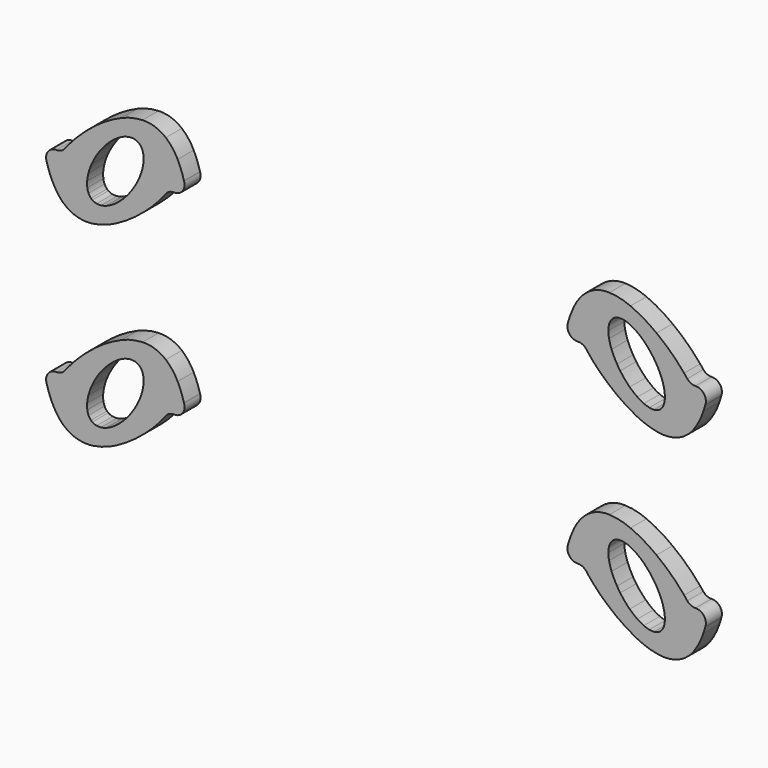
from build123d import *

# Parameters (mm, degrees)
F1_DEPTH = 12.7


# Not quite as in the source:
# - ends of sketch curves that miss each other by under 0.0002 mm in the source are joined


with BuildPart() as f1:
    # F0 (on Front) → F1 (new body)
    with BuildSketch(Plane.XZ):
        with BuildLine():
            ThreePointArc((-177.6953938627, 96.2951726391), (-186.946967119, 88.4805061313), (-195.2020417923, 79.6196730731))
            Line((-195.2020417923, 79.6196730731), (-197.2011042, 77.1213088))
            ThreePointArc((-197.2011042, 77.1213088), (-199.5136578752, 75.3159529873), (-202.3909333919, 74.7428131786))
            ThreePointArc((-202.3909333919, 74.7428131786), (-207.7133187116, 72.1927198012), (-208.6383219414, 66.3638994003))
            Line((-208.6383219414, 66.3638994003), (-208.5382926, 66.0395936))
            ThreePointArc((-208.5382926, 66.0395936), (-207.972327333, 64.1185028331), (-207.353315885, 62.2138423713))
            ThreePointArc((-207.353315885, 62.2138423713), (-204.7701961443, 55.9663745774), (-201.2342339233, 50.2044021579))
            ThreePointArc((-201.2342339233, 50.2044021579), (-196.8863760333, 45.6616875081), (-191.4694434874, 42.4684149565))
            Line((-191.4694434874, 42.4684149565), (-191.284098, 42.3952924))
            ThreePointArc((-191.284098, 42.3952924), (-185.1027368685, 40.9837502599), (-178.7669800767, 41.2283522882))
            ThreePointArc((-178.7669800767, 41.2283522882), (-171.6181643219, 43.0302257906), (-164.8462206323, 45.9445209219))
            ThreePointArc((-164.8462206323, 45.9445209219), (-155.3582667886, 51.6671412258), (-146.6297283987, 58.4922616416))
            ThreePointArc((-146.6297283987, 58.4922616416), (-139.9244707914, 64.8347082096), (-133.9056606053, 71.8319248327))
            Line((-133.9056606053, 71.8319248327), (-133.2299342, 72.7382086))
            ThreePointArc((-133.2299342, 72.7382086), (-130.8614812662, 74.6793213027), (-127.8599677834, 75.2862607769))
            ThreePointArc((-127.8599677834, 75.2862607769), (-122.5270410705, 77.7851692011), (-121.5411283463, 83.5914271061))
            Line((-121.5411283463, 83.5914271061), (-121.6296272, 83.8884276))
            ThreePointArc((-121.6296272, 83.8884276), (-123.378440433, 89.2760477142), (-125.6424834839, 94.468245494))
            ThreePointArc((-125.6424834839, 94.468245494), (-128.8762830329, 99.7114239774), (-133.1072855129, 104.1888096209))
            ThreePointArc((-133.1072855129, 104.1888096209), (-140.0332321267, 108.0332940551), (-147.8805780907, 109.1140330857))
            ThreePointArc((-147.8805780907, 109.1140330857), (-154.6765471368, 108.1634211001), (-161.1886536518, 105.9997872024))
            ThreePointArc((-161.1886536518, 105.9997872024), (-169.7449307333, 101.6626983872), (-177.6953938627, 96.2951726391))
        make_face()
        with BuildLine():
            ThreePointArc((-176.9480341869, 53.1001419638), (-178.3700174028, 53.5041929641), (-179.6704836172, 54.2071019928))
            ThreePointArc((-179.6704836172, 54.2071019928), (-180.120026778, 54.5527599218), (-180.5373020377, 54.9367507345))
            ThreePointArc((-180.5373020377, 54.9367507345), (-181.3997214321, 55.9967169239), (-182.0537255517, 57.1965381674))
            ThreePointArc((-182.0537255517, 57.1965381674), (-182.5422088404, 58.5758677997), (-182.8412153057, 60.0082653866))
            ThreePointArc((-182.8412153057, 60.0082653866), (-182.996770745, 61.812213744), (-182.9585847837, 63.6224550888))
            ThreePointArc((-182.9585847837, 63.6224550888), (-182.6792234379, 65.9600035096), (-182.1897058816, 68.2627290379))
            ThreePointArc((-182.1897058816, 68.2627290379), (-181.2724223103, 71.2729875245), (-180.1069387677, 74.1961219073))
            ThreePointArc((-180.1069387677, 74.1961219073), (-178.0007024043, 78.3577185897), (-175.5048634466, 82.2980118343))
            ThreePointArc((-175.5048634466, 82.2980118343), (-174.4173435256, 83.792470291), (-173.2758101811, 85.2460890182))
            ThreePointArc((-173.2758101811, 85.2460890182), (-170.6569263411, 88.2024335216), (-167.7913192063, 90.920303724))
            ThreePointArc((-167.7913192063, 90.920303724), (-165.5649042541, 92.6984257891), (-163.19628366, 94.2821808259))
            ThreePointArc((-163.19628366, 94.2821808259), (-161.2999842726, 95.3190481003), (-159.3137266172, 96.1710013699))
            ThreePointArc((-159.3137266172, 96.1710013699), (-157.7154103749, 96.6676730685), (-156.0708086919, 96.9784499128))
            ThreePointArc((-156.0708086919, 96.9784499128), (-154.6610921749, 97.057810869), (-153.2552179199, 96.9269846745))
            ThreePointArc((-153.2552179199, 96.9269846745), (-151.8332434746, 96.5229429708), (-150.5327847695, 95.8200418883))
            ThreePointArc((-150.5327847695, 95.8200418883), (-150.0832461196, 95.4743903416), (-149.6659744937, 95.0904067336))
            ThreePointArc((-149.6659744937, 95.0904067336), (-148.8035282211, 94.0304381711), (-148.1495164134, 92.8305978145))
            ThreePointArc((-148.1495164134, 92.8305978145), (-147.6610428325, 91.4512658888), (-147.3620363785, 90.0188700866))
            ThreePointArc((-147.3620363785, 90.0188700866), (-147.2065050667, 88.2149193747), (-147.2446935639, 86.4046789413))
            ThreePointArc((-147.2446935639, 86.4046789413), (-147.5240277621, 84.0671284904), (-148.0135453184, 81.7644029621))
            ThreePointArc((-148.0135453184, 81.7644029621), (-148.9308288897, 78.7541444755), (-150.0963124323, 75.8310100927))
            ThreePointArc((-150.0963124323, 75.8310100927), (-152.2025628964, 71.6694333025), (-154.6983928041, 67.7291491159))
            ThreePointArc((-154.6983928041, 67.7291491159), (-155.7859116303, 66.2346900702), (-156.927443836, 64.7810706787))
            ThreePointArc((-156.927443836, 64.7810706787), (-159.5463306489, 61.8247178881), (-162.4119445698, 59.1068427459))
            ThreePointArc((-162.4119445698, 59.1068427459), (-164.6383679218, 57.3287348477), (-167.0069856984, 55.7449809851))
            ThreePointArc((-167.0069856984, 55.7449809851), (-168.9032728768, 54.7081064054), (-170.8895245828, 53.8561560301))
            ThreePointArc((-170.8895245828, 53.8561560301), (-172.487848721, 53.3594569655), (-174.1324674845, 53.0486788344))
            ThreePointArc((-174.1324674845, 53.0486788344), (-175.5421719045, 52.9693209022), (-176.9480341869, 53.1001419638))
        make_face(mode=Mode.SUBTRACT)
    extrude(amount=F1_DEPTH)


with BuildPart() as f1b:
    # F0 (on Front) → F1, piece 2 (new body)
    with BuildSketch(Plane.XZ):
        with BuildLine():
            Line((197.2011042, -46.6997796), (195.2020734, -44.2014102))
            ThreePointArc((195.2020734, -44.2014102), (186.9469729749, -35.3405878466), (177.6953938627, -27.5259157609))
            ThreePointArc((177.6953938627, -27.5259157609), (169.7449307333, -22.1583900128), (161.1886562004, -17.8212952927))
            ThreePointArc((161.1886562004, -17.8212952927), (154.6765477311, -15.6576674389), (147.8805787114, -14.7070678147))
            ThreePointArc((147.8805787114, -14.7070678147), (140.033241985, -15.7877910583), (133.1072927899, -19.6322572713))
            ThreePointArc((133.1072927899, -19.6322572713), (128.8762888916, -24.1096567935), (125.6424960866, -29.3528491583))
            ThreePointArc((125.6424960866, -29.3528491583), (123.3784626535, -34.5450490683), (121.629632462, -39.9326622292))
            Line((121.629632462, -39.9326622292), (121.5411336, -40.229663))
            ThreePointArc((121.5411336, -40.229663), (122.5270410705, -46.0359191989), (127.8599678166, -48.5348283769))
            ThreePointArc((127.8599678166, -48.5348283769), (130.8614904645, -49.141771462), (133.2299305689, -51.0829079075))
            Line((133.2299305689, -51.0829079075), (133.9056758, -51.9891518))
            ThreePointArc((133.9056758, -51.9891518), (139.9244908242, -58.9863745636), (146.6297484323, -65.3288331002))
            ThreePointArc((146.6297484323, -65.3288331002), (155.3582746235, -72.153952571), (164.8462212522, -77.8765664355))
            ThreePointArc((164.8462212522, -77.8765664355), (171.6181672262, -80.7908549881), (178.7669774619, -82.5927513887))
            ThreePointArc((178.7669774619, -82.5927513887), (185.1027368685, -82.8373381401), (191.2840912155, -81.4257777575))
            Line((191.2840912155, -81.4257777575), (191.4694418, -81.3526694))
            ThreePointArc((191.4694418, -81.3526694), (196.8863760333, -78.1594008919), (201.2342450386, -73.6166943298))
            ThreePointArc((201.2342450386, -73.6166943298), (204.7701906585, -67.854724589), (207.3533009369, -61.6072664326))
            ThreePointArc((207.3533009369, -61.6072664326), (207.9723237758, -59.7025970512), (208.5382965738, -57.7814959111))
            Line((208.5382965738, -57.7814959111), (208.6383432, -57.4571876))
            ThreePointArc((208.6383432, -57.4571876), (207.7133441116, -51.6283685988), (202.390958682, -49.0782722124))
            ThreePointArc((202.390958682, -49.0782722124), (199.5136608193, -48.505162162), (197.2011042, -46.6997796))
        make_face()
        with BuildLine():
            ThreePointArc((181.6418108826, -67.4343387272), (180.7757849638, -68.6323663846), (179.6704878904, -69.6139923518))
            ThreePointArc((179.6704878904, -69.6139923518), (179.1919244089, -69.9182129674), (178.6883710607, -70.1789938892))
            ThreePointArc((178.6883710607, -70.1789938892), (177.3973595426, -70.6268807263), (176.046206417, -70.8310787354))
            ThreePointArc((176.046206417, -70.8310787354), (174.582987936, -70.8183379879), (173.1347072073, -70.6094026153))
            ThreePointArc((173.1347072073, -70.6094026153), (171.3863477646, -70.1385669414), (169.6983350536, -69.4835393235))
            ThreePointArc((169.6983350536, -69.4835393235), (167.5973067728, -68.4215563874), (165.6008854485, -67.1739866994))
            ThreePointArc((165.6008854485, -67.1739866994), (163.0858995952, -65.2824509498), (160.7376709293, -63.1874846573))
            ThreePointArc((160.7376709293, -63.1874846573), (157.5474251459, -59.7849217056), (154.6983881005, -56.091942552))
            ThreePointArc((154.6983881005, -56.091942552), (153.666026198, -54.5588585969), (152.6904970156, -52.9889990603))
            ThreePointArc((152.6904970156, -52.9889990603), (150.8081304363, -49.5169353174), (149.2342629952, -45.8945772719))
            ThreePointArc((149.2342629952, -45.8945772719), (148.3248710619, -43.1942704045), (147.6467445575, -40.4268180092))
            ThreePointArc((147.6467445575, -40.4268180092), (147.3209800199, -38.2902606469), (147.1997449811, -36.1324142807))
            ThreePointArc((147.1997449811, -36.1324142807), (147.2796619641, -34.4606010377), (147.5501168773, -32.8088736105))
            ThreePointArc((147.5501168773, -32.8088736105), (147.9577088343, -31.4570460365), (148.5614749513, -30.1807113181))
            ThreePointArc((148.5614749513, -30.1807113181), (149.4274916362, -28.9826784154), (150.5327887096, -28.0010524482))
            ThreePointArc((150.5327887096, -28.0010524482), (151.0113422017, -27.6968375795), (151.5148846236, -27.4360605956))
            ThreePointArc((151.5148846236, -27.4360605956), (152.8059065439, -26.9881666685), (154.1570716534, -26.7839659792))
            ThreePointArc((154.1570716534, -26.7839659792), (155.6202894054, -26.7967068686), (157.0685693927, -27.0056421847))
            ThreePointArc((157.0685693927, -27.0056421847), (158.8169128719, -27.4764726285), (160.5049109204, -28.1314916634))
            ThreePointArc((160.5049109204, -28.1314916634), (162.6059551987, -29.1934801671), (164.6023911515, -30.4410581006))
            ThreePointArc((164.6023911515, -30.4410581006), (167.1173770048, -32.3325938502), (169.4656056707, -34.4275601427))
            ThreePointArc((169.4656056707, -34.4275601427), (172.6558467449, -37.8301175616), (175.5048801864, -41.5230903297))
            ThreePointArc((175.5048801864, -41.5230903297), (176.5372520953, -43.05616342), (177.5127795844, -44.6260203397))
            ThreePointArc((177.5127795844, -44.6260203397), (179.3951308102, -48.0981047048), (180.9689999614, -51.7204727638))
            ThreePointArc((180.9689999614, -51.7204727638), (181.8784020662, -54.4207624375), (182.556527143, -57.1882023739))
            ThreePointArc((182.556527143, -57.1882023739), (182.8822978837, -59.3247712766), (183.0035318338, -61.4826303007))
            ThreePointArc((183.0035318338, -61.4826303007), (182.9236130271, -63.1544336228), (182.6531585177, -64.8061511889))
            ThreePointArc((182.6531585177, -64.8061511889), (182.2455712306, -66.1579897591), (181.6418108826, -67.4343387272))
        make_face(mode=Mode.SUBTRACT)
    extrude(amount=F1_DEPTH)


with BuildPart() as f1c:
    # F0 (on Front) → F1, piece 3 (new body)
    with BuildSketch(Plane.XZ):
        with BuildLine():
            Line((197.2011042, 77.1213088), (195.202048, 79.6196782))
            ThreePointArc((195.202048, 79.6196782), (186.946967119, 88.4805061313), (177.6953938627, 96.2951726391))
            ThreePointArc((177.6953938627, 96.2951726391), (169.7449307333, 101.6626983872), (161.1886562004, 105.9997931073))
            ThreePointArc((161.1886562004, 105.9997931073), (154.6765471368, 108.1634211001), (147.8805774921, 109.114020644))
            ThreePointArc((147.8805774921, 109.114020644), (140.0332321267, 108.0332940551), (133.1072777232, 104.1888186512))
            ThreePointArc((133.1072777232, 104.1888186512), (128.8762830329, 99.7114239774), (125.6424960866, 94.4682392417))
            ThreePointArc((125.6424960866, 94.4682392417), (123.378440433, 89.2760477142), (121.6296088071, 83.8884325957))
            Line((121.6296088071, 83.8884325957), (121.5411336, 83.5914254))
            ThreePointArc((121.5411336, 83.5914254), (122.5270410705, 77.7851692011), (127.8599678166, 75.2862600231))
            ThreePointArc((127.8599678166, 75.2862600231), (130.8614812662, 74.6793213027), (133.229918397, 72.7381968166))
            Line((133.229918397, 72.7381968166), (133.9056758, 71.8319366))
            ThreePointArc((133.9056758, 71.8319366), (139.9244707914, 64.8347082096), (146.6297230323, 58.4922552998))
            ThreePointArc((146.6297230323, 58.4922552998), (155.3582667886, 51.6671412258), (164.8462212522, 45.9445219645))
            ThreePointArc((164.8462212522, 45.9445219645), (171.6181643219, 43.0302257906), (178.7669767587, 41.2283328438))
            ThreePointArc((178.7669767587, 41.2283328438), (185.1027368685, 40.9837502599), (191.2840912155, 42.3953106425))
            Line((191.2840912155, 42.3953106425), (191.4694418, 42.468419))
            ThreePointArc((191.4694418, 42.468419), (196.8863760333, 45.6616875081), (201.2342450386, 50.2043940702))
            ThreePointArc((201.2342450386, 50.2043940702), (204.7701961443, 55.9663745774), (207.3533083756, 62.2138449609))
            ThreePointArc((207.3533083756, 62.2138449609), (207.972327333, 64.1185028331), (208.5382965738, 66.0395924889))
            Line((208.5382965738, 66.0395924889), (208.6383178, 66.3639008))
            ThreePointArc((208.6383178, 66.3639008), (207.7133187116, 72.1927198012), (202.390933282, 74.7428161876))
            ThreePointArc((202.390933282, 74.7428161876), (199.5136578752, 75.3159529873), (197.2011042, 77.1213088))
        make_face()
        with BuildLine():
            ThreePointArc((181.6418108826, 56.3867496728), (180.7757849638, 55.1887220154), (179.6704878904, 54.2070960482))
            ThreePointArc((179.6704878904, 54.2070960482), (179.1919134729, 53.9028945411), (178.6883613761, 53.6421154265))
            ThreePointArc((178.6883613761, 53.6421154265), (177.3973576804, 53.1942134829), (176.0462063316, 52.9900111351))
            ThreePointArc((176.0462063316, 52.9900111351), (174.582987936, 53.0027504121), (173.1347072073, 53.2116857847))
            ThreePointArc((173.1347072073, 53.2116857847), (171.3863451709, 53.6825139865), (169.6983307601, 54.3375395569))
            ThreePointArc((169.6983307601, 54.3375395569), (167.5973067728, 55.3995320126), (165.6008854485, 56.6471017006))
            ThreePointArc((165.6008854485, 56.6471017006), (163.0858995952, 58.5386374502), (160.7376709293, 60.6336037427))
            ThreePointArc((160.7376709293, 60.6336037427), (157.5474251459, 64.0361666944), (154.6983881005, 67.729145848))
            ThreePointArc((154.6983881005, 67.729145848), (153.6660082898, 69.2622182257), (152.6904782782, 70.8320781665))
            ThreePointArc((152.6904782782, 70.8320781665), (150.8081304363, 74.3041530826), (149.2342629952, 77.9265111281))
            ThreePointArc((149.2342629952, 77.9265111281), (148.3248710619, 80.6268179955), (147.6467445575, 83.3942703908))
            ThreePointArc((147.6467445575, 83.3942703908), (147.3209548909, 85.5308251494), (147.1997195829, 87.6886739026))
            ThreePointArc((147.1997195829, 87.6886739026), (147.2796619641, 89.3604873623), (147.5501168773, 91.0122147895))
            ThreePointArc((147.5501168773, 91.0122147895), (147.957686674, 92.3640507825), (148.5614557429, 93.6403879874))
            ThreePointArc((148.5614557429, 93.6403879874), (149.4274916362, 94.8384099846), (150.5327887096, 95.8200359518))
            ThreePointArc((150.5327887096, 95.8200359518), (151.0113468271, 96.1242534816), (151.5148943083, 96.3850322888))
            ThreePointArc((151.5148943083, 96.3850322888), (152.805911638, 96.8329229888), (154.1570716534, 97.0371224208))
            ThreePointArc((154.1570716534, 97.0371224208), (155.6202770217, 97.0243824743), (157.0685451022, 96.8154514068))
            ThreePointArc((157.0685451022, 96.8154514068), (158.8169010671, 96.3446196392), (160.5049109204, 95.6895967366))
            ThreePointArc((160.5049109204, 95.6895967366), (162.6059551987, 94.6276082329), (164.6023911515, 93.3800302994))
            ThreePointArc((164.6023911515, 93.3800302994), (167.1173894145, 91.4885097773), (169.4656183649, 89.3935413416))
            ThreePointArc((169.4656183649, 89.3935413416), (172.6558252148, 85.9909662917), (175.5048511812, 82.2980032389))
            ThreePointArc((175.5048511812, 82.2980032389), (176.5372464439, 80.7649337135), (177.5127795844, 79.1950680603))
            ThreePointArc((177.5127795844, 79.1950680603), (179.3951288175, 75.7229877857), (180.968996701, 72.1006241323))
            ThreePointArc((180.968996701, 72.1006241323), (181.8784007951, 69.4003303401), (182.556527143, 66.6328860261))
            ThreePointArc((182.556527143, 66.6328860261), (182.8822978837, 64.4963171234), (183.0035318338, 62.3384580993))
            ThreePointArc((183.0035318338, 62.3384580993), (182.9235879044, 60.6666574083), (182.6531343227, 59.0149426105))
            ThreePointArc((182.6531343227, 59.0149426105), (182.2455628115, 57.6631021621), (181.6418108826, 56.3867496728))
        make_face(mode=Mode.SUBTRACT)
    extrude(amount=F1_DEPTH)


with BuildPart() as f1d:
    # F0 (on Front) → F1, piece 4 (new body)
    with BuildSketch(Plane.XZ):
        with BuildLine():
            ThreePointArc((-177.6953938627, -27.5259157609), (-186.9469729749, -35.3405878466), (-195.2020520922, -44.2014277981))
            Line((-195.2020520922, -44.2014277981), (-197.2011042, -46.6997796))
            ThreePointArc((-197.2011042, -46.6997796), (-199.5136608193, -48.505162162), (-202.3909596842, -49.0782996615))
            ThreePointArc((-202.3909596842, -49.0782996615), (-207.7133441116, -51.6283685988), (-208.6383473414, -57.4571889997))
            Line((-208.6383473414, -57.4571889997), (-208.5382926, -57.7814948))
            ThreePointArc((-208.5382926, -57.7814948), (-207.9723237758, -59.7025970512), (-207.3533081368, -61.6072687912))
            ThreePointArc((-207.3533081368, -61.6072687912), (-204.7701906585, -67.854724589), (-201.2342339233, -73.6166862421))
            ThreePointArc((-201.2342339233, -73.6166862421), (-196.8863760333, -78.1594008919), (-191.4694434874, -81.3526734435))
            Line((-191.4694434874, -81.3526734435), (-191.284098, -81.425796))
            ThreePointArc((-191.284098, -81.425796), (-185.1027368685, -82.8373381401), (-178.7669800767, -82.5927361118))
            ThreePointArc((-178.7669800767, -82.5927361118), (-171.6181672262, -80.7908549881), (-164.8462261767, -77.8765569859))
            ThreePointArc((-164.8462261767, -77.8765569859), (-155.3582746235, -72.153952571), (-146.6297426525, -65.328839363))
            ThreePointArc((-146.6297426525, -65.328839363), (-139.9244908242, -58.9863745636), (-133.9056764828, -51.9891512712))
            Line((-133.9056764828, -51.9891512712), (-133.2299342, -51.0829052))
            ThreePointArc((-133.2299342, -51.0829052), (-130.8614904645, -49.141771462), (-127.8599677834, -48.5348276231))
            ThreePointArc((-127.8599677834, -48.5348276231), (-122.5270410705, -46.0359191989), (-121.5411283463, -40.2296612939))
            Line((-121.5411283463, -40.2296612939), (-121.6296272, -39.9326608))
            ThreePointArc((-121.6296272, -39.9326608), (-123.3784626535, -34.5450490683), (-125.6425038809, -29.3528530078))
            ThreePointArc((-125.6425038809, -29.3528530078), (-128.8762888916, -24.1096567935), (-133.1073000843, -19.6322662178))
            ThreePointArc((-133.1073000843, -19.6322662178), (-140.033241985, -15.7877910583), (-147.8805793101, -14.707055373))
            ThreePointArc((-147.8805793101, -14.707055373), (-154.6765477311, -15.6576674389), (-161.1886536518, -17.8213011976))
            ThreePointArc((-161.1886536518, -17.8213011976), (-169.7449307333, -22.1583900128), (-177.6953938627, -27.5259157609))
        make_face()
        with BuildLine():
            ThreePointArc((-176.9480341869, -70.7209464362), (-178.3700174028, -70.3168954359), (-179.6704836172, -69.6139864072))
            ThreePointArc((-179.6704836172, -69.6139864072), (-180.1200373693, -69.2683409431), (-180.5373148061, -68.8843503653))
            ThreePointArc((-180.5373148061, -68.8843503653), (-181.3997418805, -67.8243788549), (-182.0537509517, -66.6245502326))
            ThreePointArc((-182.0537509517, -66.6245502326), (-182.5422101983, -65.245215752), (-182.8412153057, -63.8128230134))
            ThreePointArc((-182.8412153057, -63.8128230134), (-182.996771564, -62.0088748281), (-182.9585828949, -60.1986334524))
            ThreePointArc((-182.9585828949, -60.1986334524), (-182.6792234379, -57.8610848904), (-182.1897058816, -55.5583593621))
            ThreePointArc((-182.1897058816, -55.5583593621), (-181.2724223103, -52.5481008755), (-180.1069387677, -49.6249664927))
            ThreePointArc((-180.1069387677, -49.6249664927), (-178.000707536, -45.4633788446), (-175.5048753963, -41.5230935661))
            ThreePointArc((-175.5048753963, -41.5230935661), (-174.4173498004, -40.0286264079), (-173.2758101811, -38.5749993818))
            ThreePointArc((-173.2758101811, -38.5749993818), (-170.6569268744, -35.6186545514), (-167.7913175603, -32.9007865699))
            ThreePointArc((-167.7913175603, -32.9007865699), (-165.5649130077, -31.1226690154), (-163.1963021863, -29.5389188588))
            ThreePointArc((-163.1963021863, -29.5389188588), (-161.2999980181, -28.5020469868), (-159.3137349454, -27.650090142))
            ThreePointArc((-159.3137349454, -27.650090142), (-157.7154146996, -27.1534164083), (-156.0708086919, -26.8426384872))
            ThreePointArc((-156.0708086919, -26.8426384872), (-154.6610921749, -26.763277531), (-153.2552179199, -26.8941037255))
            ThreePointArc((-153.2552179199, -26.8941037255), (-151.8332475972, -27.2981540807), (-150.5327929828, -28.0010583928))
            ThreePointArc((-150.5327929828, -28.0010583928), (-150.0832461196, -28.3466980584), (-149.6659744937, -28.7306816664))
            ThreePointArc((-149.6659744937, -28.7306816664), (-148.8035282211, -29.7906502289), (-148.1495164134, -30.9904905855))
            ThreePointArc((-148.1495164134, -30.9904905855), (-147.6610428325, -32.3698225112), (-147.3620363785, -33.8022183134))
            ThreePointArc((-147.3620363785, -33.8022183134), (-147.2065050667, -35.6061690253), (-147.2446935639, -37.4164094587))
            ThreePointArc((-147.2446935639, -37.4164094587), (-147.5240530093, -39.7539589873), (-148.0135707184, -42.0566854379))
            ThreePointArc((-148.0135707184, -42.0566854379), (-148.9308299465, -45.0669469353), (-150.0963124323, -47.9900783073))
            ThreePointArc((-150.0963124323, -47.9900783073), (-152.2025628964, -52.1516550975), (-154.6983928041, -56.0919392841))
            ThreePointArc((-154.6983928041, -56.0919392841), (-155.7859116303, -57.5863983298), (-156.927443836, -59.0400177213))
            ThreePointArc((-156.927443836, -59.0400177213), (-159.5463306489, -61.9963705119), (-162.4119445698, -64.7142456541))
            ThreePointArc((-162.4119445698, -64.7142456541), (-164.6383679218, -66.4923535523), (-167.0069856984, -68.0761074149))
            ThreePointArc((-167.0069856984, -68.0761074149), (-168.903267884, -69.1129926088), (-170.8895193665, -69.9649463297))
            ThreePointArc((-170.8895193665, -69.9649463297), (-172.487848721, -70.4616314345), (-174.1324674845, -70.7724095656))
            ThreePointArc((-174.1324674845, -70.7724095656), (-175.5421719045, -70.8517674978), (-176.9480341869, -70.7209464362))
        make_face(mode=Mode.SUBTRACT)
    extrude(amount=F1_DEPTH)


solid = Compound([f1.part, f1b.part, f1c.part, f1d.part])
